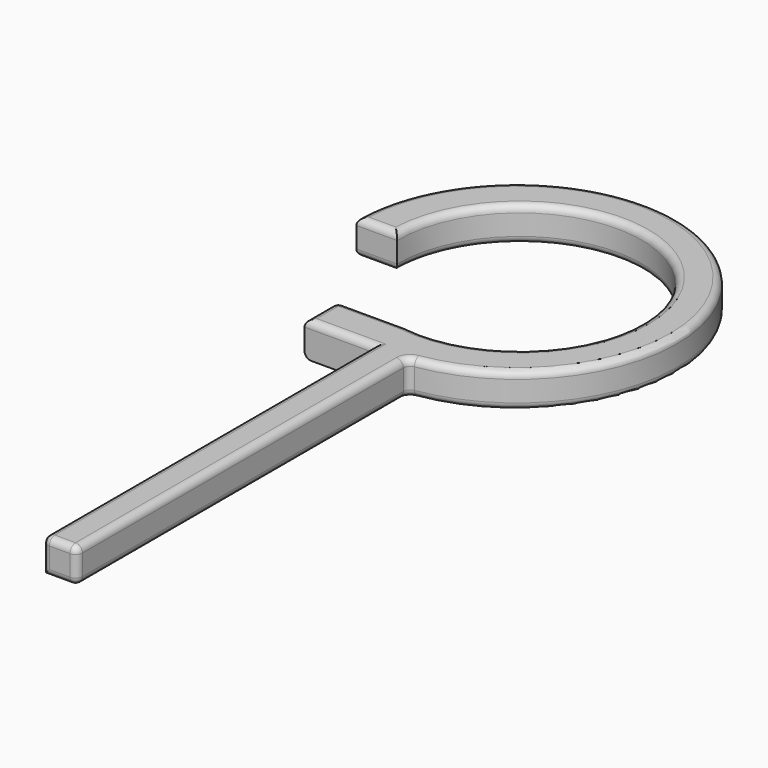
from build123d import *

# Parameters (mm, degrees)
F0_W     = 12.7
F0_H     = 7.493
F1_DEPTH = 6.35
F2_R     = 1.27


# Not quite as in the source:
# - two fillets or chamfers of one size are made in one step
# - a feature names something its author has since deleted; it is built from what else it names


with BuildPart() as f1:
    # F0 (on Top) → F1 (new body)
    with BuildSketch(Plane.XY):
        with BuildLine():
            Line((-2.8947171572, -21.8944355268), (-2.8947171572, -29.3874355268))
            ThreePointArc((-2.8947171572, -29.3874355268), (0.2819172587, -29.5283131405), (3.4552828428, -29.3268098289))
            ThreePointArc((3.4552828428, -29.3268098289), (19.6210018926, 22.0684625426), (-29.5296588918, 0))
            Line((-29.5296588918, 0), (-22.0366588918, 0))
            ThreePointArc((-22.0366588918, 0), (17.2330212266, 15.017871009), (-2.8947171572, -21.8944355268))
        make_face()
        with BuildLine():
            ThreePointArc((3.4552828428, -29.3268098289), (0.2819172587, -29.5283131405), (-2.8947171572, -29.3874355268))
            Line((-2.8947171572, -29.3874355268), (-2.8947171572, -105.5874355268))
            Line((-2.8947171572, -105.5874355268), (3.4552828428, -105.5874355268))
            Line((3.4552828428, -105.5874355268), (3.4552828428, -29.3268098289))
        make_face()
        with Locations((-9.2447171572, -25.6409355268)):
            Rectangle(F0_W, F0_H)
    extrude(amount=F1_DEPTH)

    # F2
    f2_edges = [f1.edges().sort_by_distance(p)[0] for p in [
        (19.621002, 22.068463, 6.35),
        (-25.783159, 0, 6.35),
        (17.233021, 15.017871, 6.35),
        (-9.244717, -21.894436, 6.35),
        (-15.594717, -25.640936, 6.35),
        (-9.244717, -29.387436, 6.35),
        (-2.894717, -67.487436, 6.35),
        (0.280283, -105.587436, 6.35),
        (3.455283, -67.457123, 6.35),
        (-15.594717, -25.640936, 0),
        (-15.594717, -21.894436, 3.175),
        (-25.783159, 0, 0),
        (17.233021, 15.017871, 0),
        (-2.894717, -105.587436, 3.175),
        (3.455283, -105.587436, 3.175),
        (0.280283, -105.587436, 0),
        (3.455283, -29.32681, 3.175),
        (3.455283, -67.457123, 0),
        (19.621002, 22.068463, 0),
    ]]
    fillet(f2_edges, radius=F2_R)


solid = f1.part
